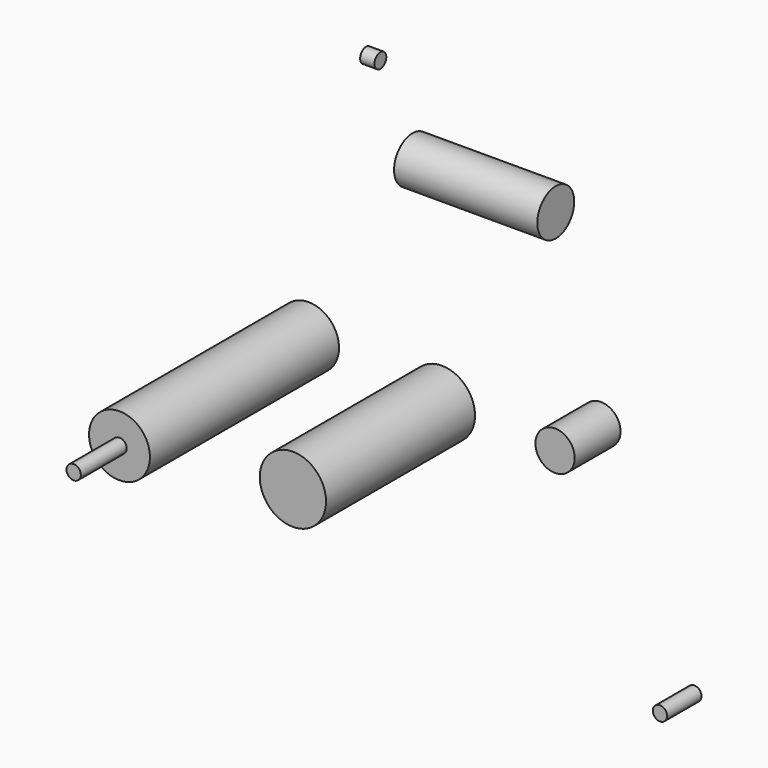
from build123d import *

# Parameters (mm, degrees)
F0_R      = 53.975
F1_DEPTH  = 419.1
F2_R      = 12.7
F3_DEPTH  = 101.6
F4_R      = 40.9136311109
F5_DEPTH  = 254
F6_R      = 13.1158886666
F7_DEPTH  = 25.4
F8_DEPTH  = 25.4
F9_R      = 12.7
F10_DEPTH = 76.2
F11_R     = 34.8034548998
F12_DEPTH = 101.6
F13_R     = 58.7360473688
F15_DEPTH = 330.2


# Not quite as in the source:
# - a feature names something its author has since deleted; it is built from what else it names
# - the program builds the solid bodies; features that only make, move or delete a surface that nothing else refers to are left out


with BuildPart() as f1:
    # F0 (on Front) → F1 (new body)
    with BuildSketch(Plane.XZ):
        Circle(F0_R)
    extrude(amount=F1_DEPTH)

    # F2 (on face) → F3 (join)
    with BuildSketch(Plane.XZ.offset(419.1)):
        Circle(F2_R)
    extrude(amount=F3_DEPTH)

    # F0 (on Front) → F8 (join)
    with BuildSketch(Plane.XZ):
        Circle(F0_R)
    extrude(amount=F8_DEPTH)


with BuildPart() as f5:
    # F4 (on Right) → F5 (new body)
    with BuildSketch(Plane.YZ):
        with Locations((230.3282767534, 183.0985844135)):
            Circle(F4_R)
    extrude(amount=F5_DEPTH)


with BuildPart() as f7:
    # F6 (on Right) → F7 (new body)
    with BuildSketch(Plane.YZ):
        with Locations((127.3537427187, 387.6445889473)):
            Circle(F6_R)
    extrude(amount=F7_DEPTH)


with BuildPart() as f10:
    # F9 (on face) → F10 (new body)
    with BuildSketch(Plane(origin=(0, 0, 0), x_dir=(-1, 0, 0), z_dir=(0, 1, 0))):
        with Locations((-623.0502128601, -385.4478597641)):
            Circle(F9_R)
    extrude(amount=F10_DEPTH)


with BuildPart() as f12:
    # F11 (on Front) → F12 (new body)
    with BuildSketch(Plane.XZ):
        with Locations((518.3054804802, 31.798414886)):
            Circle(F11_R)
    extrude(amount=F12_DEPTH)


with BuildPart() as f15:
    # F13 (on Front) → F15 (new body)
    with BuildSketch(Plane.XZ):
        with Locations((236.3598048687, -27.1700881422)):
            Circle(F13_R)
    extrude(amount=F15_DEPTH)


solid = Compound([f1.part, f5.part, f7.part, f10.part, f12.part, f15.part])
